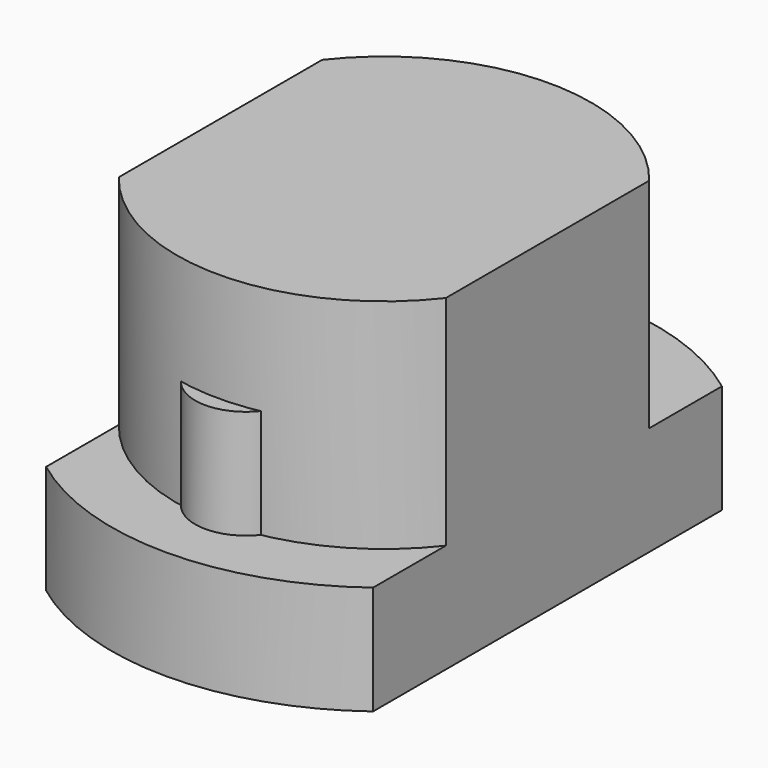
from build123d import *

# Parameters (mm, degrees)
F0_R      = 12.5
F1_DEPTH  = 5
F2_R      = 9.5
F3_DEPTH  = 10
F5_DEPTH  = 5
F7_W      = 30
F7_H      = 30
F7_W_2    = 15
F7_H_2    = 27
F8_DEPTH  = 10
F11_W     = 23.265004158
F11_H     = 35.2036263794
F12_DEPTH = 35


# Not quite as in the source:
# - a feature names something its author has since deleted; it is built from what else it names


with BuildPart() as f1:
    # F0 (on Top) → F1 (new body)
    with BuildSketch(Plane.XY):
        Circle(F0_R)
    extrude(amount=-F1_DEPTH)

    # F2 (on Top) → F3 (join)
    with BuildSketch(Plane.XY):
        Circle(F2_R)
    extrude(amount=F3_DEPTH)


with BuildPart() as f5:
    # F4 (on Top) → F5 (new body)
    with BuildSketch(Plane.XY):
        with BuildLine():
            ThreePointArc((-2.19192449, 8.7487287819), (-0.0332522533, 9.0190732649), (2.1273547272, 8.7646534521))
            ThreePointArc((2.1273547272, 8.7646534521), (-0.0376344683, 10.2076699565), (-2.19192449, 8.7487287819))
        make_face()
    extrude(amount=F5_DEPTH)


with BuildPart() as f6_1:
    # F6: instance of F5
    add(f5.part.mirror(Plane.XZ))


with BuildPart() as f8:
    # F7 (on Top) → F8 (new body, symmetric)
    with BuildSketch(Plane.XY):
        Rectangle(F7_W, F7_H)
        Rectangle(F7_W_2, F7_H_2, mode=Mode.SUBTRACT)
    extrude(amount=F8_DEPTH, both=True)


with BuildPart() as f1_1:
    add(f1.part)

    # F9: cut F8
    add(f8.part, mode=Mode.SUBTRACT)


with BuildPart() as f12:
    # F11 (on face) → F12 (new body)
    with BuildSketch(Plane(origin=(0, 0, -5), x_dir=(1, 0, 0), z_dir=(0, 0, -1))):
        with Locations((0.5739731714, -1.2244740501)):
            Rectangle(F11_W, F11_H)
        with BuildLine():
            Line((-7, 10.3561575886), (-7, 13.5))
            Line((-7, 13.5), (7, 13.5))
            Line((7, 13.5), (7, 10.3561575886))
            ThreePointArc((7, 10.3561575886), (7.2521867086, 10.1811486554), (7.5, 10))
            Line((7.5, 10), (7.5, -10))
            ThreePointArc((7.5, -10), (7.2521867086, -10.1811486554), (7, -10.3561575886))
            Line((7, -10.3561575886), (7, -13.5))
            Line((7, -13.5), (-7, -13.5))
            Line((-7, -13.5), (-7, -10.3561575886))
            ThreePointArc((-7, -10.3561575886), (-7.2521867086, -10.1811486554), (-7.5, -10))
            Line((-7.5, -10), (-7.5, 10))
            ThreePointArc((-7.5, 10), (-7.2521867086, 10.1811486554), (-7, 10.3561575886))
        make_face(mode=Mode.SUBTRACT)
    extrude(amount=-F12_DEPTH)


with BuildPart() as f6_1_1:
    add(f6_1.part)

    # F13: cut F12
    add(f12.part, mode=Mode.SUBTRACT)


with BuildPart() as f5_1:
    add(f5.part)

    # F13: cut F12
    add(f12.part, mode=Mode.SUBTRACT)


with BuildPart() as f1_2:
    add(f1_1.part)

    # F13: cut F12
    add(f12.part, mode=Mode.SUBTRACT)


solid = Compound([f6_1_1.part, f5_1.part, f1_2.part])
